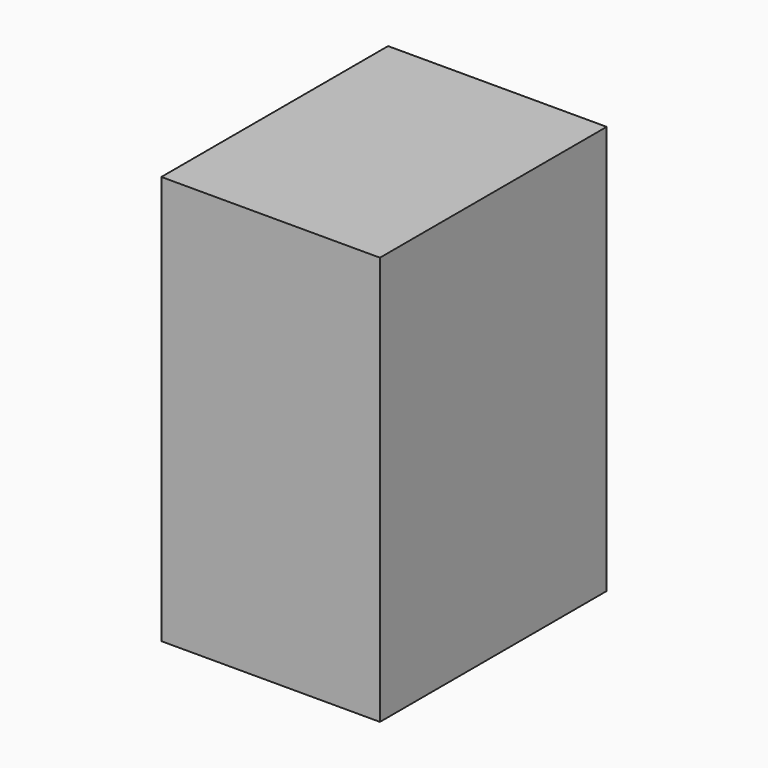
from build123d import *

# Parameters (mm, degrees)
F0_W     = 67.9279565811
F0_H     = 88.0647003651
F1_DEPTH = 127


# Not quite as in the source:
# - a feature of the source that left no trace in its solid (it failed there, or was rolled back) is left out


with BuildPart() as f1:
    # F0 (on Top) → F1 (new body)
    with BuildSketch(Plane.XY):
        Rectangle(F0_W, F0_H)
    extrude(amount=-F1_DEPTH)


solid = f1.part
